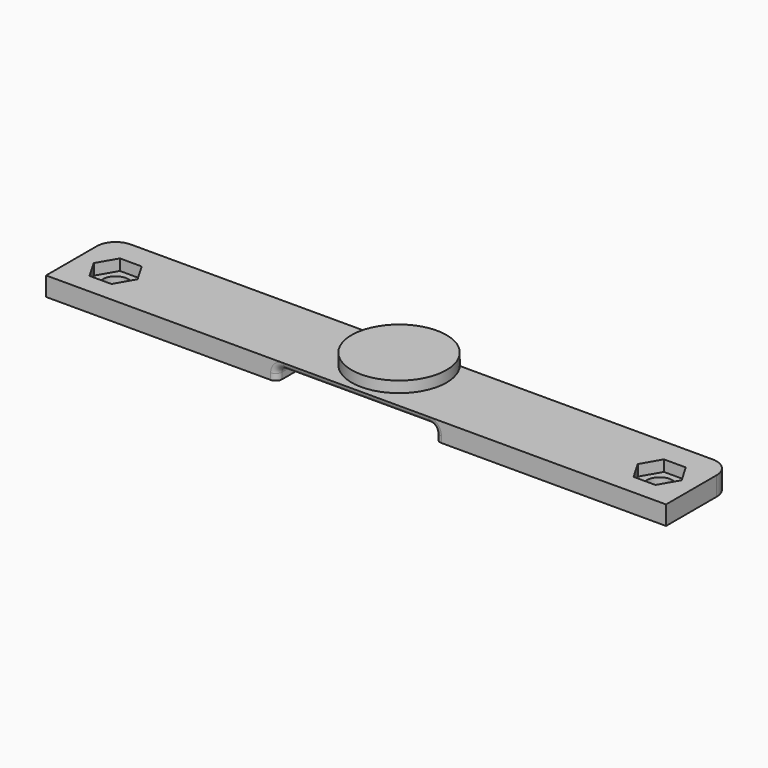
from build123d import *

# Parameters (mm, degrees)
F0_W      = 98
F0_H      = 13
F1_DEPTH  = 3
F2_R      = 3
F3_R      = 2
F4_DEPTH  = 20
F5_R      = 7.5
F6_DEPTH  = 4.75
F8_DEPTH  = 1.75
F9_W      = 25
F9_H      = 16
F10_DEPTH = 2
F11_F1_R  = 1
F11_F2_R  = 0.9999


# Not quite as in the source:
# - a fillet or chamfer is up to 0.001 mm smaller than in the source, because OpenCascade refuses the exact size


with BuildPart() as f1:
    # F0 (on Top) → F1 (new body)
    with BuildSketch(Plane.XY):
        with Locations((5.7567551136, -20.2820947109)):
            Rectangle(F0_W, F0_H)
    extrude(amount=F1_DEPTH)

    # F2
    f2_edges = [f1.edges().sort_by_distance(p)[0] for p in [
        (-43.243245, -13.782095, 1.5),
        (54.756755, -13.782095, 1.5),
    ]]
    fillet(f2_edges, radius=F2_R)

    # F3 (on face) → F4 (cut)
    with BuildSketch(Plane.XY.offset(3)):
        with Locations((48.7567551136, -20.5320947109)):
            Circle(F3_R)
        with Locations((-37.2432448864, -20.5320947109)):
            Circle(F3_R)
    extrude(amount=-F4_DEPTH, mode=Mode.SUBTRACT)

    # F5 (on Top) → F6 (join)
    with BuildSketch(Plane.XY):
        with Locations((5.7567551136, -18.2820947109)):
            Circle(F5_R)
    extrude(amount=F6_DEPTH)

    # F7 (on face) → F8 (cut)
    with BuildSketch(Plane.XY.offset(3)):
        Polygon((-33.7791432713, -20.5320947109), (-35.5111940788, -17.5320947109), (-38.975295694, -17.5320947109), (-40.7073465015, -20.5320947109), (-38.975295694, -23.5320947109), (-35.5111940788, -23.5320947109), align=None)
        Polygon((50.4888059212, -17.5320947109), (47.024704306, -17.5320947109), (45.2926534985, -20.5320947109), (47.024704306, -23.5320947109), (50.4888059212, -23.5320947109), (52.2208567287, -20.5320947109), align=None)
    extrude(amount=-F8_DEPTH, mode=Mode.SUBTRACT)

    # F9 (on face) → F10 (cut)
    with BuildSketch(Plane(origin=(0, 0, 0), x_dir=(1, 0, 0), z_dir=(0, 0, -1))):
        with Locations((5.7567551136, 18.7820947109)):
            Rectangle(F9_W, F9_H)
    extrude(amount=-F10_DEPTH, mode=Mode.SUBTRACT)

    # F11: fillet of radius 1 on 6 edges, made by hand

    # F11_f1
    f11_f1_edges = [f1.edges().sort_by_distance(p)[0] for p in [
        (18.2567551136, -20.2820947109, 2),
        (-6.7432448864, -20.2820947109, 2),
    ]]
    fillet(f11_f1_edges, radius=F11_F1_R)

    # F11_f2 (radius 1 in the source; OpenCascade refuses exactly that, so slightly less here)
    f11_f2_edges = [f1.edges().sort_by_distance(p)[0] for p in [
        (14.5067551136, -13.7820947109, 2),
        (5.7567551136, -10.7820947109, 2),
        (-2.9932448864, -13.7820947109, 2),
        (5.7567551136, -26.7820947109, 2),
        (17.9638618948, -26.7820947109, 1.7071067812),
        (-6.4503516676, -26.7820947109, 1.7071067812),
        (-6.4503516676, -13.7820947109, 1.7071067812),
        (17.9638618948, -13.7820947109, 1.7071067812),
    ]]
    fillet(f11_f2_edges, radius=F11_F2_R)


solid = f1.part
